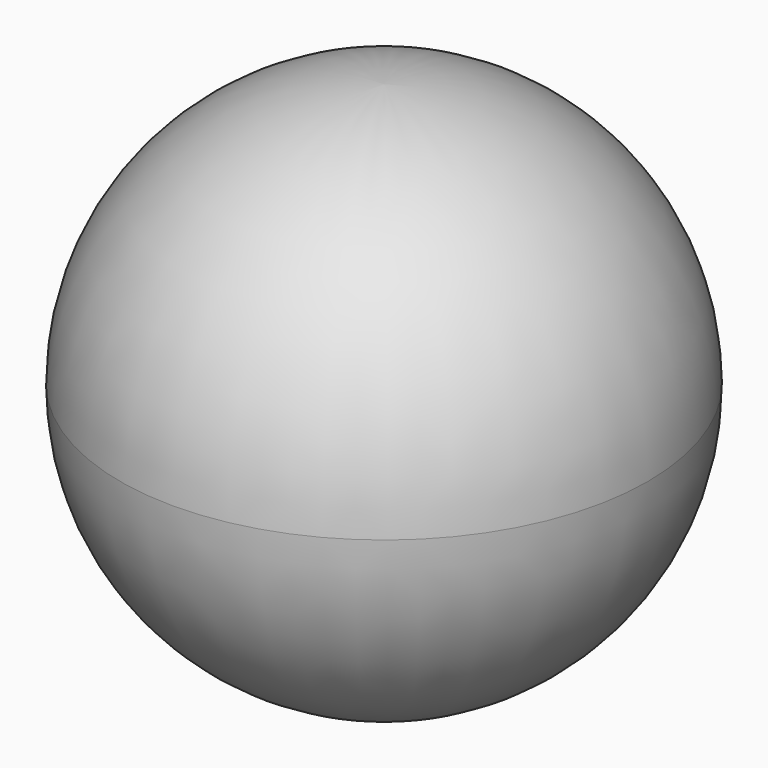
from build123d import *

# Parameters (mm, degrees)
F0_R     = 15
F1_DEPTH = 15
F2_R     = 14.99999


# Not quite as in the source:
# - a fillet or chamfer is up to 0.001 mm smaller than in the source, because OpenCascade refuses the exact size


with BuildPart() as f1:
    # F0 (on Top) → F1 (new body, symmetric)
    with BuildSketch(Plane.XY):
        Circle(F0_R)
    extrude(amount=F1_DEPTH, both=True)

    # F2 (radius 15 in the source; OpenCascade refuses exactly that, so slightly less here)
    f2_edges = [f1.edges().sort_by_distance(p)[0] for p in [
        (-15, 0, 15),
        (-15, 0, -15),
    ]]
    fillet(f2_edges, radius=F2_R)


solid = f1.part
